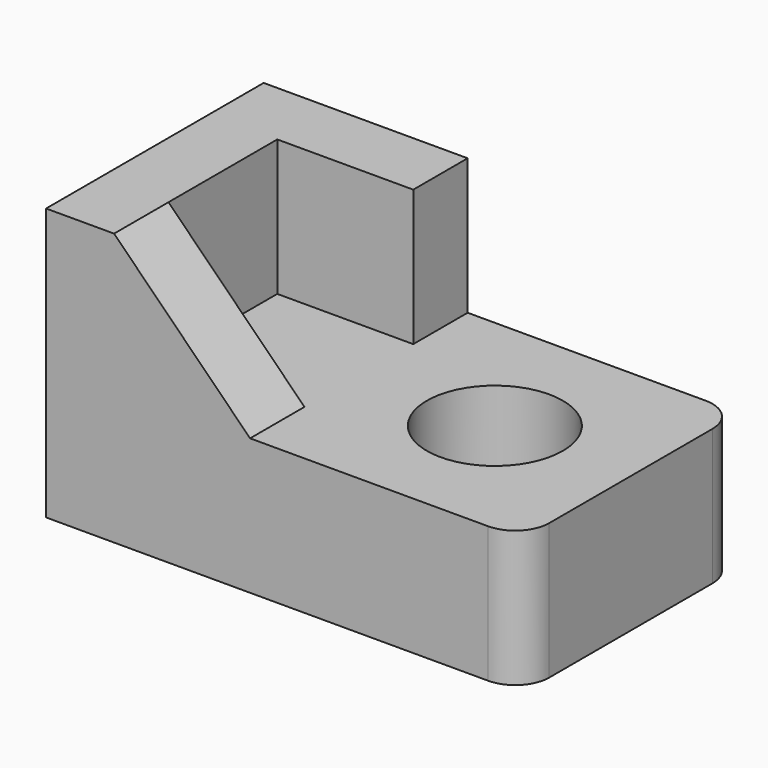
from build123d import *

# Parameters (mm, degrees)
F0_R     = 10
F1_DEPTH = 20
F2_DEPTH = 40
F3_SIZE  = 19.99999


# Not quite as in the source:
# - a fillet or chamfer is up to 0.001 mm smaller than in the source, because OpenCascade refuses the exact size


with BuildPart() as f1:
    # F0 (on Top) → F1 (new body)
    with BuildSketch(Plane.XY):
        with BuildLine():
            Line((15, 20), (-20, 20))
            Line((-20, 20), (-20, 10))
            Line((-20, 10), (-40, 10))
            Line((-40, 10), (-40, -10))
            Line((-40, -10), (-20, -10))
            Line((-20, -10), (-20, -20))
            Line((-20, -20), (15, -20))
            ThreePointArc((15, -20), (18.5355339059, -18.5355339059), (20, -15))
            Line((20, -15), (20, 15))
            ThreePointArc((20, 15), (18.5355339059, 18.5355339059), (15, 20))
        make_face()
        Circle(F0_R, mode=Mode.SUBTRACT)
    extrude(amount=F1_DEPTH)

    # F0 (on Top) → F2 (join)
    with BuildSketch(Plane.XY):
        Polygon((-40, 20), (-50, 20), (-50, 10), (-50, -10), (-50, -20), (-40, -20), (-20, -20), (-20, -10), (-40, -10), (-40, 10), (-20, 10), (-20, 20), align=None)
    extrude(amount=F2_DEPTH)

    # F3 (size 20 in the source; OpenCascade refuses exactly that, so slightly less here)
    f3_edges = [f1.edges().sort_by_distance(p)[0] for p in [
        (-20, -15, 40),
    ]]
    chamfer(f3_edges, length=F3_SIZE)


solid = f1.part
